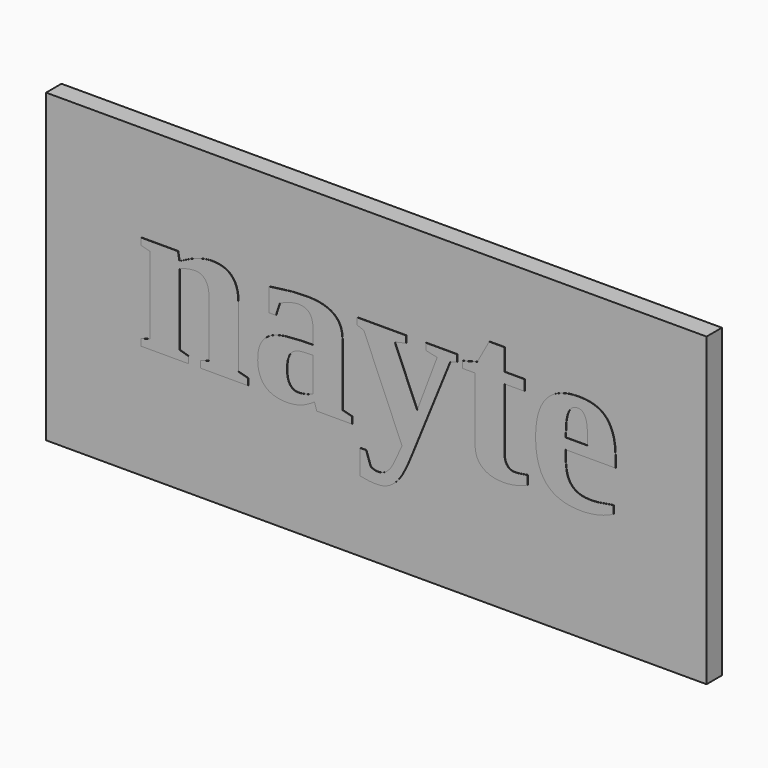
from build123d import *

# Parameters (mm, degrees)
F0_TEXT_SIZE = 38.474377964
F1_DEPTH     = 3.64911
F2_W         = 122.0555901527
F2_H         = 56.5669750795
F3_DEPTH     = 3.556


# Not quite as in the source:
# - Text() gives the source's letters only with a copy of the font that has no kerning and outlines rounded to 1/6400 em; it was checked with that copy


with BuildPart() as f1:
    # F0 (on Front) → F1 (new body)
    with BuildSketch(Plane.XZ):
        with Locations((-44.3807961436, 15.8626127897)):
            Text('nayte', F0_TEXT_SIZE, font='Tinos', font_style=FontStyle.BOLD, text_align=(TextAlign.LEFT, TextAlign.BOTTOM))
    extrude(amount=F1_DEPTH)


with BuildPart() as f3:
    # F2 (on Front) → F3 (new body)
    with BuildSketch(Plane.XZ):
        with Locations((0.0949092209, 23.0633807369)):
            Rectangle(F2_W, F2_H)
    extrude(amount=F3_DEPTH)


solid = Compound([f1.part, f3.part])
